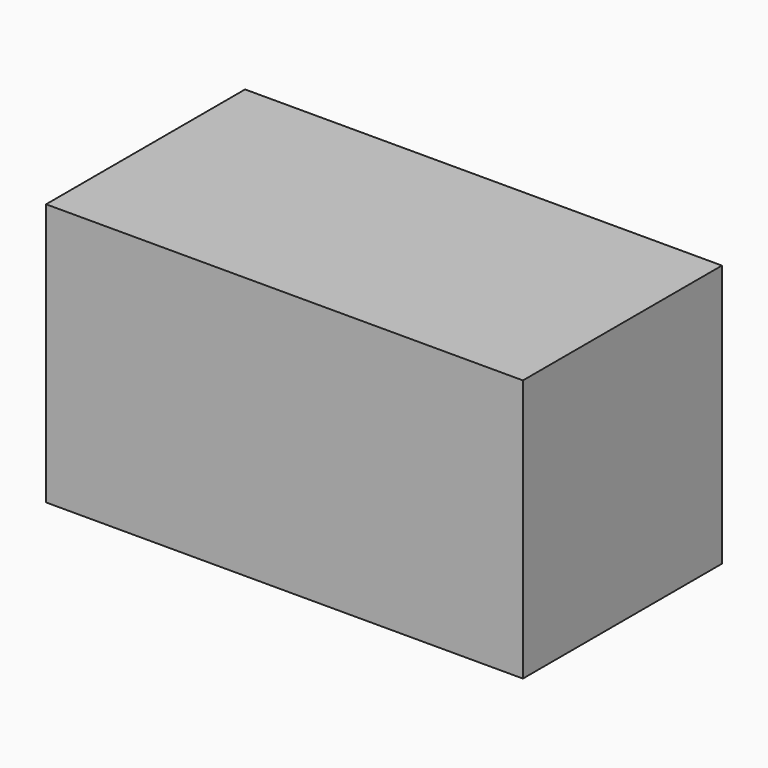
from build123d import *

# Parameters (mm, degrees)
F0_W     = 48.6929183826
F0_H     = 26.8050543964
F1_DEPTH = 25.4


# Not quite as in the source:
# - the program builds the solid bodies; features that only make, move or delete a surface that nothing else refers to are left out


with BuildPart() as f1:
    # F0 (on Front) → F1 (new body)
    with BuildSketch(Plane.XZ):
        with Locations((-39.1043764539, 44.7071250528)):
            Rectangle(F0_W, F0_H)
    extrude(amount=F1_DEPTH)


solid = f1.part
